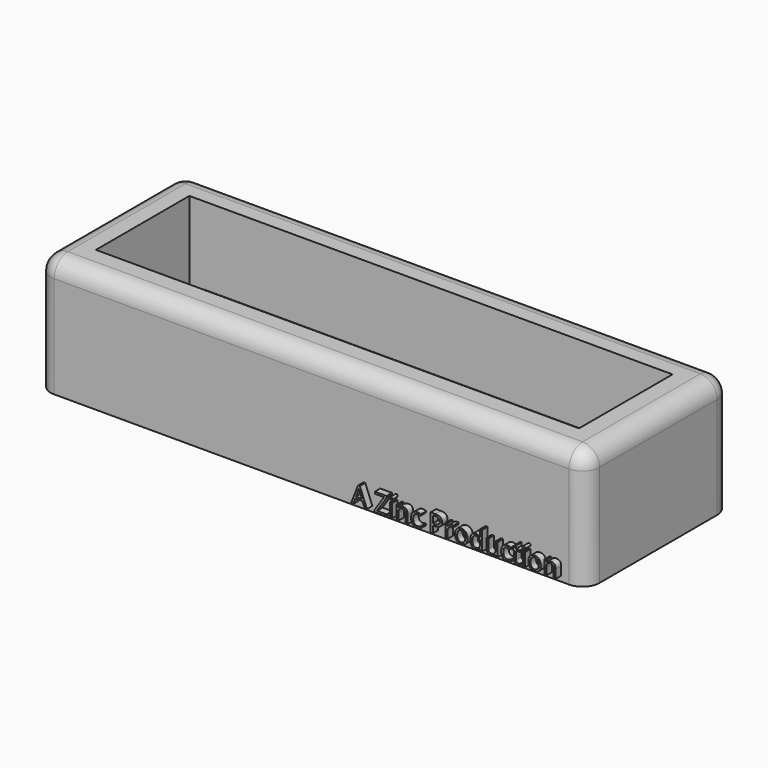
from build123d import *

# Parameters (mm, degrees)
F0_W          = 164.3055900931
F0_H          = 54.2125031352
F1_DEPTH      = 35.56
F2_R          = 5.08
F3_W          = 144.6863897145
F3_H          = 34.9920894951
F4_DEPTH      = 27.94
F5_TEXT_SIZE  = 7.5410654991
F6_DEPTH      = 2.032
F7_W          = 128.325175494
F7_H          = 26.3471193612
F8_DEPTH      = 7.874
F9_W          = 123.8962374628
F9_H          = 21.971788723
F10_DEPTH     = 13.462
F11_TEXT_SIZE = 20.571191433
F12_DEPTH     = 9.652


# Not quite as in the source:
# - Text() gives the source's letters only with a copy of the font that has no kerning and outlines rounded to 1/6400 em; it was checked with that copy


with BuildPart() as f1:
    # F0 (on Top) → F1 (new body)
    with BuildSketch(Plane.XY):
        with Locations((-25.2873040736, -6.9662444293)):
            Rectangle(F0_W, F0_H)
    extrude(amount=F1_DEPTH)

    # F2
    f2_edges = [f1.edges().sort_by_distance(p)[0] for p in [
        (-107.440099, -6.966244, 35.56),
        (-25.287304, 20.140007, 35.56),
        (56.865491, -6.966244, 35.56),
        (-25.287304, -34.072496, 35.56),
        (56.865491, -34.072496, 17.78),
        (56.865491, 20.140007, 17.78),
        (-107.440099, -34.072496, 17.78),
        (-107.440099, 20.140007, 17.78),
    ]]
    fillet(f2_edges, radius=F2_R)

    # F3 (on face) → F4 (cut)
    with BuildSketch(Plane.XY.offset(35.56)):
        with Locations((-25.449289009, -6.6838832572)):
            Rectangle(F3_W, F3_H)
    extrude(amount=-F4_DEPTH, mode=Mode.SUBTRACT)

    # F5 (on face) → F6 (join)
    with BuildSketch(Plane.XZ.offset(34.072495997)):
        with Locations((-11.8624595925, 1.5535714615)):
            Text('A Zinc Production', F5_TEXT_SIZE, font='Open Sans', text_align=(TextAlign.LEFT, TextAlign.BOTTOM))
    extrude(amount=F6_DEPTH)

    # F7 (on face) → F8 (join)
    with BuildSketch(Plane.XY.offset(7.62)):
        with Locations((-25.3801513463, -7.1325916797)):
            Rectangle(F7_W, F7_H)
    extrude(amount=F8_DEPTH)

    # F9 (on face) → F10 (cut)
    with BuildSketch(Plane.XY.offset(15.494)):
        with Locations((-25.480972603, -7.2221884038)):
            Rectangle(F9_W, F9_H)
    extrude(amount=-F10_DEPTH, mode=Mode.SUBTRACT)

    # F11 (on face) → F12 (join)
    with BuildSketch(Plane.XY.offset(2.032)):
        with Locations((-42.1799495816, -14.8112578318)):
            Text('Z T', F11_TEXT_SIZE, font='Open Sans', text_align=(TextAlign.LEFT, TextAlign.BOTTOM))
    extrude(amount=F12_DEPTH)


solid = f1.part
